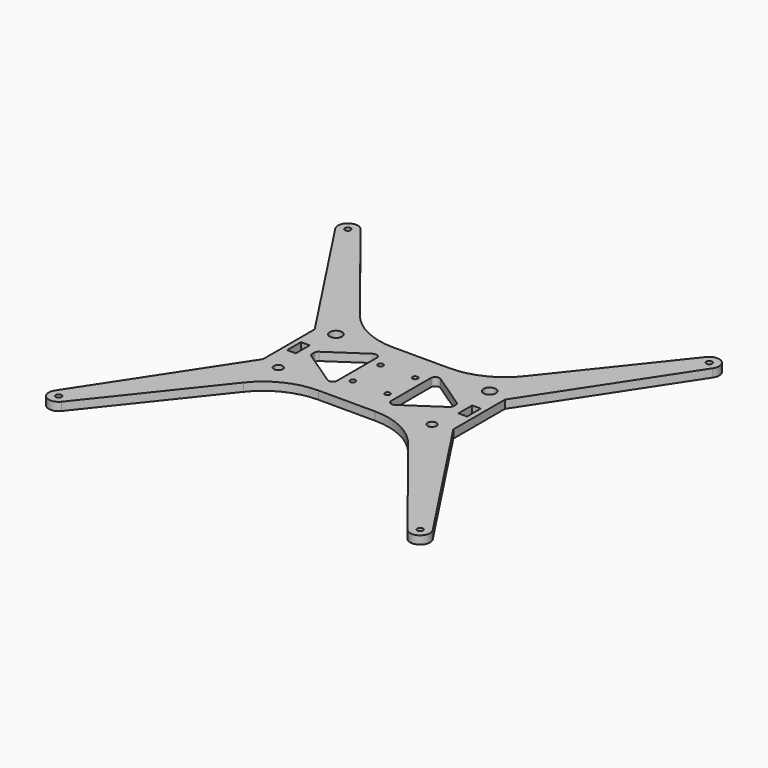
from build123d import *

# Parameters (mm, degrees)
F0_R     = 1.65
F0_R_2   = 2.55
F0_W     = 5
F0_H     = 10
F0_R_3   = 1.5
F0_R_4   = 3.555
F1_DEPTH = 4.75


# Not quite as in the source:
# - ends of sketch curves that miss each other by under 0.0002 mm in the source are joined


with BuildPart() as f1:
    # F0 (on Top) → F1 (new body)
    with BuildSketch(Plane.XY):
        with BuildLine():
            Line((-47.640397, 42.115595), (-100.031737, 108.050449))
            ThreePointArc((-100.031737, 108.050449), (-107.8442155419, 109.1246397394), (-109.2715048598, 101.368896092))
            Line((-109.2715048598, 101.368896092), (-54.999977, 18.664241))
            Line((-54.999977, 18.664241), (-54.999977, -18.664242))
            Line((-54.999977, -18.664242), (-109.271505, -101.368897))
            ThreePointArc((-109.271505, -101.368897), (-107.8441644553, -109.1246766812), (-100.031658534, -108.0503513703))
            Line((-100.031658534, -108.0503513703), (-47.643302, -42.116283))
            ThreePointArc((-47.643302, -42.116283), (-33.7130803066, -30.9767526972), (-16.325566, -27))
            Line((-16.325566, -27), (16.325565, -27))
            ThreePointArc((16.325565, -27), (33.7130793066, -30.9767526972), (47.6433013924, -42.1162826882))
            Line((47.6433013924, -42.1162826882), (100.031658, -108.050351))
            ThreePointArc((100.031658, -108.050351), (107.8441644255, -109.1246767027), (109.2715050175, -101.3688963323))
            Line((109.2715050175, -101.3688963323), (54.999976, -18.664242))
            Line((54.999976, -18.664242), (54.999976, 18.664241))
            Line((54.999976, 18.664241), (109.271504, 101.368896))
            ThreePointArc((109.271504, 101.368896), (107.8442155121, 109.1246397609), (100.0317360662, 108.0504489474))
            Line((100.0317360662, 108.0504489474), (47.640396, 42.115595))
            ThreePointArc((47.640396, 42.115595), (33.7103248028, 30.9765618002), (16.323206, 27))
            Line((16.323206, 27), (-16.323206, 27))
            ThreePointArc((-16.323206, 27), (-33.710325083, 30.9765619354), (-47.640397, 42.115595))
        make_face()
        with Locations((-104.5, -104.5)):
            Circle(F0_R, mode=Mode.SUBTRACT)
        with Locations((-44.444977, -20.807752)):
            Circle(F0_R_2, mode=Mode.SUBTRACT)
        with Locations((-49.499977, 0)):
            Rectangle(F0_W, F0_H, mode=Mode.SUBTRACT)
        with BuildLine():
            Line((-19.581953, -16.373154), (-39.803759, -2.743263))
            ThreePointArc((-39.803759, -2.743263), (-40.6136447533, -1.8442487652), (-40.906473, -0.670199))
            Line((-40.906473, -0.670199), (-40.906473, 0.670176))
            ThreePointArc((-40.906473, 0.670176), (-40.6136450793, 1.8442251525), (-39.8037598701, 2.7432388072))
            Line((-39.8037598701, 2.7432388072), (-19.581955, 16.373149))
            ThreePointArc((-19.581955, 16.373149), (-17.0106188475, 16.5072580793), (-15.684668, 14.300086))
            Line((-15.684668, 14.300086), (-15.684668, -14.30009))
            ThreePointArc((-15.684668, -14.30009), (-17.0106178687, -16.5072615586), (-19.581953, -16.373154))
        make_face(mode=Mode.SUBTRACT)
        with Locations((-10, -10)):
            Circle(F0_R_3, mode=Mode.SUBTRACT)
        with Locations((104.5, -104.5)):
            Circle(F0_R, mode=Mode.SUBTRACT)
        with Locations((10, -10)):
            Circle(F0_R_3, mode=Mode.SUBTRACT)
        with Locations((44.444976, -20.807752)):
            Circle(F0_R_2, mode=Mode.SUBTRACT)
        with BuildLine():
            Line((19.581954, 16.373149), (39.803759, 2.743239))
            ThreePointArc((39.803759, 2.743239), (40.6136440793, 1.8442251525), (40.906472, 0.670176))
            Line((40.906472, 0.670176), (40.906472, -0.670199))
            ThreePointArc((40.906472, -0.670199), (40.6136437533, -1.8442487652), (39.803757719, -2.7432625831))
            Line((39.803757719, -2.7432625831), (19.581952, -16.373154))
            ThreePointArc((19.581952, -16.373154), (17.0106168687, -16.5072615586), (15.684667, -14.30009))
            Line((15.684667, -14.30009), (15.684667, 14.300086))
            ThreePointArc((15.684667, 14.300086), (17.0106178475, 16.5072580793), (19.581954, 16.373149))
        make_face(mode=Mode.SUBTRACT)
        with Locations((49.499976, 0)):
            Rectangle(F0_W, F0_H, mode=Mode.SUBTRACT)
        with Locations((-44.444977, 20.810818)):
            Circle(F0_R_4, mode=Mode.SUBTRACT)
        with Locations((-10, 10)):
            Circle(F0_R_3, mode=Mode.SUBTRACT)
        with Locations((-104.5, 104.5)):
            Circle(F0_R, mode=Mode.SUBTRACT)
        with Locations((10, 10)):
            Circle(F0_R_3, mode=Mode.SUBTRACT)
        with Locations((44.444976, 20.810818)):
            Circle(F0_R_4, mode=Mode.SUBTRACT)
        with Locations((104.5, 104.5)):
            Circle(F0_R, mode=Mode.SUBTRACT)
    extrude(amount=F1_DEPTH)


solid = f1.part
